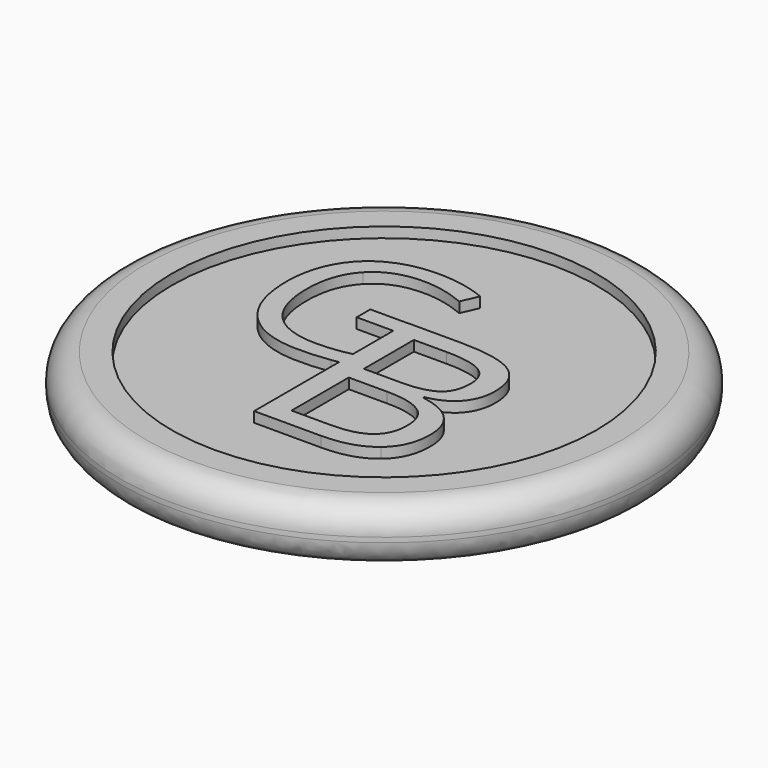
from build123d import *

# Parameters (mm, degrees)
F0_R         = 51
F1_DEPTH     = 10
F2_R         = 41
F3_DEPTH     = 2
F4_W         = 7.0717344974
F4_H         = 3.2909496187
F5_DEPTH     = 2
F6_R         = 5
F7_SIZE      = 2
F8_R         = 5
F9_TEXT_SIZE = 13.8888888889
F10_DEPTH    = 2


# Not quite as in the source:
# - Text() gives the source's letters only with a copy of the font that has no kerning and outlines rounded to 1/6400 em; it was checked with that copy


with BuildPart() as f1:
    # F0 (on Top) → F1 (new body)
    with BuildSketch(Plane.XY):
        Circle(F0_R)
    extrude(amount=F1_DEPTH)

    # F2 (on face) → F3 (cut)
    with BuildSketch(Plane.XY.offset(10)):
        Circle(F2_R)
    extrude(amount=-F3_DEPTH, mode=Mode.SUBTRACT)

    # F4 (on face) → F5 (join)
    with BuildSketch(Plane.XY.offset(8)):
        with Locations((-6.760397643, 7.8990585806)):
            Rectangle(F4_W, F4_H)
        with BuildLine():
            Line((-3.2245303943, 9.5817206029), (-3.2245303943, 9.54453339))
            Line((-3.2245303943, 9.54453339), (0.4634082828, 9.54453339))
            Line((0.4634082828, 9.54453339), (0.4634082828, -5.8501825107))
            add(Edge.make_bspline(
                [(0.4634082828, -5.8501825107), (-1.3587398994, -6.4324667783), (-3.2245303943, -6.8092684905)],
                knots=[0, 0, 0, 0.7245184394, 0.7245184394, 0.7245184394], degree=2))
            Line((-3.2245303943, -6.8092684905), (-3.2245303943, -27.3496636655))
            Line((-3.2245303943, -27.3496636655), (9.6598264724, -27.3496636655))
            add(Edge.make_bspline(
                [(19.0199803316, -24.5690998248), (15.6736040814, -27.3496636655), (9.6598264724, -27.3496636655)],
                knots=[0, 0, 0, 1, 1, 1], degree=2))
            add(Edge.make_bspline(
                [(22.3663565818, -16.8417189185), (22.3663565818, -21.788535984), (19.0199803316, -24.5690998248)],
                knots=[0, 0, 0, 1, 1, 1], degree=2))
            add(Edge.make_bspline(
                [(13.9519177498, -7.9988792622), (22.3663565818, -9.4376593891), (22.3663565818, -16.8417189185)],
                knots=[0, 0, 0, 1, 1, 1], degree=2))
            Line((13.9519177498, -7.9988792622), (13.9519177498, -7.7483051952))
            add(Edge.make_bspline(
                [(19.2988450191, -4.9839074233), (17.4680377228, -7.1178285104), (13.9519177498, -7.7483051952)],
                knots=[0, 0, 0, 1, 1, 1], degree=2))
            add(Edge.make_bspline(
                [(21.1296523154, 0.439808673), (21.1296523154, -2.8499863362), (19.2988450191, -4.9839074233)],
                knots=[0, 0, 0, 1, 1, 1], degree=2))
            add(Edge.make_bspline(
                [(17.8438988234, 7.3831352405), (21.1296523154, 5.184549878), (21.1296523154, 0.439808673)],
                knots=[0, 0, 0, 1, 1, 1], degree=2))
            add(Edge.make_bspline(
                [(7.2106670429, 9.5817206029), (14.5581453313, 9.5817206029), (17.8438988234, 7.3831352405)],
                knots=[0, 0, 0, 1, 1, 1], degree=2))
            Line((7.2106670429, 9.5817206029), (-3.2245303943, 9.5817206029))
        make_face()
        with BuildLine():
            Line((1.0675608831, -23.6880490729), (1.0675608831, -9.8660602134))
            Line((1.0675608831, -9.8660602134), (8.423122206, -9.8660602134))
            add(Edge.make_bspline(
                [(15.455362152, -11.4826670976), (13.1436143077, -9.8660602134), (8.423122206, -9.8660602134)],
                knots=[0, 0, 0, 1, 1, 1], degree=2))
            add(Edge.make_bspline(
                [(17.7671099964, -16.5345636105), (17.7671099964, -13.0992739817), (15.455362152, -11.4826670976)],
                knots=[0, 0, 0, 1, 1, 1], degree=2))
            add(Edge.make_bspline(
                [(15.5079018758, -21.9582797069), (17.7671099964, -20.2285103408), (17.7671099964, -16.5345636105)],
                knots=[0, 0, 0, 1, 1, 1], degree=2))
            add(Edge.make_bspline(
                [(8.7787757205, -23.6880490729), (13.2486937552, -23.6880490729), (15.5079018758, -21.9582797069)],
                knots=[0, 0, 0, 1, 1, 1], degree=2))
            Line((8.7787757205, -23.6880490729), (1.0675608831, -23.6880490729))
        make_face(mode=Mode.SUBTRACT)
        with BuildLine():
            Line((8.1402160013, -6.2286947241), (1.0675608831, -6.2286947241))
            Line((1.0675608831, -6.2286947241), (1.0675608831, 5.8635247694))
            Line((1.0675608831, 5.8635247694), (7.3884938001, 5.8635247694))
            add(Edge.make_bspline(
                [(14.4611489183, 4.4894089178), (12.2383144526, 5.8635247694), (7.3884938001, 5.8635247694)],
                knots=[0, 0, 0, 1, 1, 1], degree=2))
            add(Edge.make_bspline(
                [(16.683983384, 0.0033248143), (16.683983384, 3.1152930663), (14.4611489183, 4.4894089178)],
                knots=[0, 0, 0, 1, 1, 1], degree=2))
            add(Edge.make_bspline(
                [(14.6874738821, -4.8020391488), (16.683983384, -3.3753835736), (16.683983384, 0.0033248143)],
                knots=[0, 0, 0, 1, 1, 1], degree=2))
            add(Edge.make_bspline(
                [(8.1402160013, -6.2286947241), (12.6909643802, -6.2286947241), (14.6874738821, -4.8020391488)],
                knots=[0, 0, 0, 1, 1, 1], degree=2))
        make_face(mode=Mode.SUBTRACT)
        with BuildLine():
            Line((0.4634082828, 9.54453339), (-3.2245303943, 9.54453339))
            Line((-3.2245303943, 9.54453339), (-3.2245303943, 6.2535837713))
            Line((-3.2245303943, 6.2535837713), (-3.2224552902, 6.2535837713))
            Line((-3.2224552902, 6.2535837713), (-3.2224552902, -3.4876271002))
            add(Edge.make_bspline(
                [(-3.2245303943, -3.4881309013), (-3.2234928339, -3.4878790424), (-3.2224552902, -3.4876271002)],
                knots=[0.9996694169, 0.9996694169, 0.9996694169, 1, 1, 1], degree=2))
            Line((-3.2245303943, -3.4881309013), (-3.2245303943, -6.8092684905))
            add(Edge.make_bspline(
                [(0.4634082828, -5.8501825107), (-1.3587398994, -6.4324667783), (-3.2245303943, -6.8092684905)],
                knots=[0, 0, 0, 0.7245184394, 0.7245184394, 0.7245184394], degree=2))
            Line((0.4634082828, -5.8501825107), (0.4634082828, 9.54453339))
        make_face()
        with BuildLine():
            Line((-3.2224552902, 6.2535837713), (-3.2245303943, 6.2535837713))
            Line((-3.2245303943, 6.2535837713), (-3.2245303943, -3.4881309013))
            add(Edge.make_bspline(
                [(-3.2245303943, -3.4881309013), (-3.2234928339, -3.4878790424), (-3.2224552902, -3.4876271002)],
                knots=[0.9996694169, 0.9996694169, 0.9996694169, 1, 1, 1], degree=2))
            Line((-3.2224552902, -3.4876271002), (-3.2224552902, 6.2535837713))
        make_face()
        with BuildLine():
            Line((-3.2245303943, -6.8092684905), (-3.2245303943, -3.4881309013))
            add(Edge.make_bspline(
                [(-9.6519315979, -4.2497417487), (-6.3620699114, -4.2497417487), (-3.2245303943, -3.4881309013)],
                knots=[0, 0, 0, 0.9996694169, 0.9996694169, 0.9996694169], degree=2))
            add(Edge.make_bspline(
                [(-18.8423414279, -0.938007185), (-15.7142072114, -4.2497417487), (-9.6519315979, -4.2497417487)],
                knots=[0, 0, 0, 1, 1, 1], degree=2))
            add(Edge.make_bspline(
                [(-21.9704756445, 8.7824187415), (-21.9704756445, 2.3737273787), (-18.8423414279, -0.938007185)],
                knots=[0, 0, 0, 1, 1, 1], degree=2))
            add(Edge.make_bspline(
                [(-18.7210959157, 18.3331009508), (-21.9704756445, 14.8931925598), (-21.9704756445, 8.7824187415)],
                knots=[0, 0, 0, 1, 1, 1], degree=2))
            add(Edge.make_bspline(
                [(-9.6935014879, 21.7730093417), (-15.4717161869, 21.7730093417), (-18.7210959157, 18.3331009508)],
                knots=[0, 0, 0, 1, 1, 1], degree=2))
            add(Edge.make_bspline(
                [(-1.4418783386, 19.9577908152), (-5.7305053154, 21.7730093417), (-9.6935014879, 21.7730093417)],
                knots=[0, 0, 0, 1, 1, 1], degree=2))
            Line((-1.4418783386, 19.9577908152), (-0.0146454513, 23.207170544))
            add(Edge.make_bspline(
                [(-9.4579387783, 25.0639589604), (-4.386412208, 25.0639589604), (-0.0146454513, 23.207170544)],
                knots=[0, 0, 0, 1, 1, 1], degree=2))
            add(Edge.make_bspline(
                [(-18.1772231892, 23.1067099767), (-14.4532538838, 25.0639589604), (-9.4579387783, 25.0639589604)],
                knots=[0, 0, 0, 1, 1, 1], degree=2))
            add(Edge.make_bspline(
                [(-23.8826905809, 17.43588416), (-21.9011924946, 21.1494609929), (-18.1772231892, 23.1067099767)],
                knots=[0, 0, 0, 1, 1, 1], degree=2))
            add(Edge.make_bspline(
                [(-25.8641886671, 8.7824187415), (-25.8641886671, 13.722307327), (-23.8826905809, 17.43588416)],
                knots=[0, 0, 0, 1, 1, 1], degree=2))
            add(Edge.make_bspline(
                [(-21.8596226047, -3.2001020282), (-25.8641886671, 1.0781324761), (-25.8641886671, 8.7824187415)],
                knots=[0, 0, 0, 1, 1, 1], degree=2))
            add(Edge.make_bspline(
                [(-10.670393901, -7.4783365326), (-17.8550565423, -7.4783365326), (-21.8596226047, -3.2001020282)],
                knots=[0, 0, 0, 1, 1, 1], degree=2))
            add(Edge.make_bspline(
                [(-4.6496881775, -7.0661017909), (-7.2478062975, -7.4783365326), (-10.670393901, -7.4783365326)],
                knots=[0, 0, 0, 1, 1, 1], degree=2))
            add(Edge.make_bspline(
                [(-3.2245303943, -6.8092684905), (-3.9339545432, -6.9525387209), (-4.6496881775, -7.0661017909)],
                knots=[0.7245184394, 0.7245184394, 0.7245184394, 1, 1, 1], degree=2))
        make_face()
    extrude(amount=F5_DEPTH)

    # F6
    f6_edges = [f1.edges().sort_by_distance(p)[0] for p in [
        (-51, 0, 10),
    ]]
    fillet(f6_edges, radius=F6_R)

    # F7
    f7_edges = [f1.edges().sort_by_distance(p)[0] for p in [
        (-51, 0, 0),
    ]]
    chamfer(f7_edges, length=F7_SIZE)

    # F8
    f8_edges = [f1.edges().sort_by_distance(p)[0] for p in [
        (-51, 0, 2),
    ]]
    fillet(f8_edges, radius=F8_R)

    # F9 (on face) → F10 (cut)
    with BuildSketch(Plane(origin=(0, 0, 0), x_dir=(1, 0, 0), z_dir=(0, 0, -1))):
        with Locations(Location((45.7725694444, -4.541760566), (0, 0, 180))):
            Text('559-978-8206', F9_TEXT_SIZE, font='Open Sans', font_style=FontStyle.BOLD, text_align=(TextAlign.LEFT, TextAlign.BOTTOM))
        with Locations(Location((45.7725694444, 14.3471283229), (0, 0, 180))):
            Text('PDGA #77904', F9_TEXT_SIZE, font='Open Sans', font_style=FontStyle.BOLD, text_align=(TextAlign.LEFT, TextAlign.BOTTOM))
    extrude(amount=-F10_DEPTH, mode=Mode.SUBTRACT)


solid = f1.part
